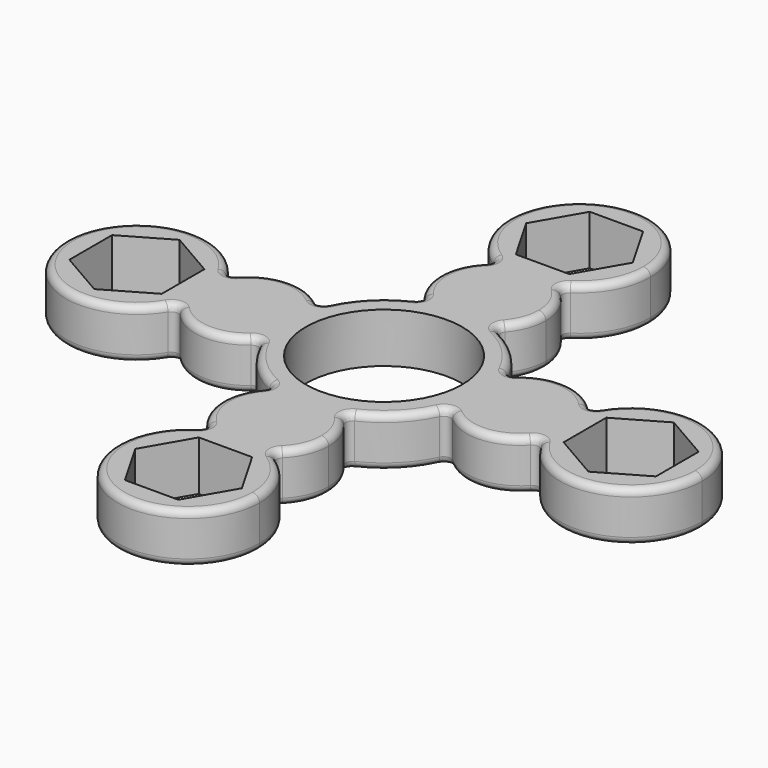
from build123d import *

# Parameters (mm, degrees)
F0_R     = 11
F1_DEPTH = 7
F2_F1_R  = 1
F2_F2_R  = 1


with BuildPart() as f1:
    # F0 (on Top) → F1 (new body)
    with BuildSketch(Plane.XY):
        with BuildLine():
            ThreePointArc((13.2109175103, -4.6337521011), (13.8013195953, -2.3502292287), (14, 0))
            ThreePointArc((14, 0), (13.8013195953, 2.3502292287), (13.2109175103, 4.6337521011))
            ThreePointArc((13.2109175103, 4.6337521011), (11.6082339734, 0), (13.2109175103, -4.6337521011))
        make_face()
        with BuildLine():
            ThreePointArc((13.2109175103, 4.6337521011), (13.8013195953, 2.3502292287), (14, 0))
            ThreePointArc((14, 0), (13.8013195953, -2.3502292287), (13.2109175103, -4.6337521011))
            ThreePointArc((13.2109175103, -4.6337521011), (19.5943342941, -7.4842305201), (25.5553991453, -3.8319787638))
            ThreePointArc((25.5553991453, -3.8319787638), (24.7920618951, 0), (25.5553991453, 3.8319787638))
            ThreePointArc((25.5553991453, 3.8319787638), (19.5943342941, 7.4842305201), (13.2109175103, 4.6337521011))
        make_face()
        with BuildLine():
            ThreePointArc((13.2109175103, -4.6337521011), (11.6082339734, 0), (13.2109175103, 4.6337521011))
            ThreePointArc((13.2109175103, 4.6337521011), (9.8975116316, 9.9014778444), (4.6284588018, 13.2127729535))
            ThreePointArc((4.6284588018, 13.2127729535), (0, 11.6142447293), (-4.6284588018, 13.2127729535))
            ThreePointArc((-4.6284588018, 13.2127729535), (-9.8975116316, 9.9014778444), (-13.2109175103, 4.6337521011))
            ThreePointArc((-13.2109175103, 4.6337521011), (-12.0202203774, 2.4515430373), (-11.6082339734, 0))
            ThreePointArc((-11.6082339734, 0), (-12.0202203774, -2.4515430373), (-13.2109175103, -4.6337521011))
            ThreePointArc((-13.2109175103, -4.6337521011), (-9.8975116316, -9.9014778444), (-4.6284588018, -13.2127729535))
            ThreePointArc((-4.6284588018, -13.2127729535), (0, -11.6142447293), (4.6284588018, -13.2127729535))
            ThreePointArc((4.6284588018, -13.2127729535), (9.8975116316, -9.9014778444), (13.2109175103, -4.6337521011))
        make_face()
        Circle(F0_R, mode=Mode.SUBTRACT)
        with BuildLine():
            ThreePointArc((-4.6284588018, 13.2127729535), (0, 11.6142447293), (4.6284588018, 13.2127729535))
            ThreePointArc((4.6284588018, 13.2127729535), (0, 14), (-4.6284588018, 13.2127729535))
        make_face()
        with BuildLine():
            ThreePointArc((-4.6284588018, 13.2127729535), (0, 14), (4.6284588018, 13.2127729535))
            ThreePointArc((4.6284588018, 13.2127729535), (6.7440136793, 15.8327390545), (7.5, 19.1142447293))
            ThreePointArc((7.5, 19.1142447293), (6.6241857963, 22.6313689147), (4.2012899905, 25.3270671487))
            ThreePointArc((4.2012899905, 25.3270671487), (0, 24.4017110765), (-4.2012899905, 25.3270671487))
            ThreePointArc((-4.2012899905, 25.3270671487), (-7.4953416797, 19.3785421075), (-4.6284588018, 13.2127729535))
        make_face()
        with BuildLine():
            ThreePointArc((44.7920618951, 0), (36.745696009, 9.8073092002), (25.5553991453, 3.8319787638))
            ThreePointArc((25.5553991453, 3.8319787638), (26.3402371118, 1.9869903385), (26.6082339734, 0))
            ThreePointArc((26.6082339734, 0), (26.3402371118, -1.9869903385), (25.5553991453, -3.8319787638))
            ThreePointArc((25.5553991453, -3.8319787638), (36.745696009, -9.8073092002), (44.7920618951, 0))
        make_face()
        Polygon((34.7920618951, 7.5055534995), (41.2920618951, 3.7527767497), (41.2920618951, -3.7527767497), (34.7920618951, -7.5055534995), (28.2920618951, -3.7527767497), (28.2920618951, 3.7527767497), align=None, mode=Mode.SUBTRACT)
        with BuildLine():
            ThreePointArc((26.6082339734, 0), (26.3402371118, 1.9869903385), (25.5553991453, 3.8319787638))
            ThreePointArc((25.5553991453, 3.8319787638), (24.7920618951, 0), (25.5553991453, -3.8319787638))
            ThreePointArc((25.5553991453, -3.8319787638), (26.3402371118, -1.9869903385), (26.6082339734, 0))
        make_face()
        with BuildLine():
            ThreePointArc((7.5, -19.1142447293), (6.7440136793, -15.8327390545), (4.6284588018, -13.2127729535))
            ThreePointArc((4.6284588018, -13.2127729535), (0, -14), (-4.6284588018, -13.2127729535))
            ThreePointArc((-4.6284588018, -13.2127729535), (-7.4953416797, -19.3785421075), (-4.2012899905, -25.3270671487))
            ThreePointArc((-4.2012899905, -25.3270671487), (0, -24.4017110765), (4.2012899905, -25.3270671487))
            ThreePointArc((4.2012899905, -25.3270671487), (6.6241857963, -22.6313689147), (7.5, -19.1142447293))
        make_face()
        with BuildLine():
            ThreePointArc((-4.6284588018, -13.2127729535), (0, -14), (4.6284588018, -13.2127729535))
            ThreePointArc((4.6284588018, -13.2127729535), (0, -11.6142447293), (-4.6284588018, -13.2127729535))
        make_face()
        with BuildLine():
            ThreePointArc((-11.6082339734, 0), (-12.0202203774, 2.4515430373), (-13.2109175103, 4.6337521011))
            ThreePointArc((-13.2109175103, 4.6337521011), (-14, 0), (-13.2109175103, -4.6337521011))
            ThreePointArc((-13.2109175103, -4.6337521011), (-12.0202203774, -2.4515430373), (-11.6082339734, 0))
        make_face()
        with BuildLine():
            ThreePointArc((-13.2109175103, -4.6337521011), (-14, 0), (-13.2109175103, 4.6337521011))
            ThreePointArc((-13.2109175103, 4.6337521011), (-19.5943342941, 7.4842305201), (-25.5553991453, 3.8319787638))
            ThreePointArc((-25.5553991453, 3.8319787638), (-24.9847526949, 1.9536341139), (-24.7920618951, 0))
            ThreePointArc((-24.7920618951, 0), (-24.9847526949, -1.9536341139), (-25.5553991453, -3.8319787638))
            ThreePointArc((-25.5553991453, -3.8319787638), (-19.5943342941, -7.4842305201), (-13.2109175103, -4.6337521011))
        make_face()
        with BuildLine():
            ThreePointArc((10, 34.4017110765), (-5.3845659108, 42.8282435753), (-4.2012899905, 25.3270671487))
            ThreePointArc((-4.2012899905, 25.3270671487), (0, 26.6142447293), (4.2012899905, 25.3270671487))
            ThreePointArc((4.2012899905, 25.3270671487), (8.4265324988, 29.0171451657), (10, 34.4017110765))
        make_face()
        Polygon((-7.5055534995, 34.4017110765), (-3.7527767497, 40.9017110765), (3.7527767497, 40.9017110765), (7.5055534995, 34.4017110765), (3.7527767497, 27.9017110765), (-3.7527767497, 27.9017110765), align=None, mode=Mode.SUBTRACT)
        with BuildLine():
            ThreePointArc((4.2012899905, 25.3270671487), (0, 26.6142447293), (-4.2012899905, 25.3270671487))
            ThreePointArc((-4.2012899905, 25.3270671487), (0, 24.4017110765), (4.2012899905, 25.3270671487))
        make_face()
        with BuildLine():
            ThreePointArc((4.2012899905, -25.3270671487), (0, -24.4017110765), (-4.2012899905, -25.3270671487))
            ThreePointArc((-4.2012899905, -25.3270671487), (0, -26.6142447293), (4.2012899905, -25.3270671487))
        make_face()
        with BuildLine():
            ThreePointArc((4.2012899905, -25.3270671487), (0, -26.6142447293), (-4.2012899905, -25.3270671487))
            ThreePointArc((-4.2012899905, -25.3270671487), (-5.3845659108, -42.8282435753), (10, -34.4017110765))
            ThreePointArc((10, -34.4017110765), (8.4265324988, -29.0171451657), (4.2012899905, -25.3270671487))
        make_face()
        Polygon((-3.7527767497, -27.9017110765), (3.7527767497, -27.9017110765), (7.5055534995, -34.4017110765), (3.7527767497, -40.9017110765), (-3.7527767497, -40.9017110765), (-7.5055534995, -34.4017110765), align=None, mode=Mode.SUBTRACT)
        with BuildLine():
            ThreePointArc((-24.7920618951, 0), (-24.9847526949, 1.9536341139), (-25.5553991453, 3.8319787638))
            ThreePointArc((-25.5553991453, 3.8319787638), (-26.6082339734, 0), (-25.5553991453, -3.8319787638))
            ThreePointArc((-25.5553991453, -3.8319787638), (-24.9847526949, -1.9536341139), (-24.7920618951, 0))
        make_face()
        with BuildLine():
            ThreePointArc((-25.5553991453, -3.8319787638), (-26.6082339734, 0), (-25.5553991453, 3.8319787638))
            ThreePointArc((-25.5553991453, 3.8319787638), (-44.7920618951, 0), (-25.5553991453, -3.8319787638))
        make_face()
        Polygon((-28.2920618951, 3.7527767497), (-28.2920618951, -3.7527767497), (-34.7920618951, -7.5055534995), (-41.2920618951, -3.7527767497), (-41.2920618951, 3.7527767497), (-34.7920618951, 7.5055534995), align=None, mode=Mode.SUBTRACT)
    extrude(amount=F1_DEPTH)

    # F2: fillet of radius 1 on 32 edges, made by hand

    # F2_f1
    f2_f1_edges = [f1.edges().sort_by_distance(p)[0] for p in [
        (-25.5553991453, -3.8319787638, 3.5),
        (-13.2109175103, -4.6337521011, 3.5),
        (4.2012899905, -25.3270671487, 3.5),
        (4.6284588018, -13.2127729535, 3.5),
        (-13.2109175103, 4.6337521011, 3.5),
        (-25.5553991453, 3.8319787638, 3.5),
        (-4.2012899905, 25.3270671487, 3.5),
        (-4.6284588018, 13.2127729535, 3.5),
        (4.6284588018, 13.2127729535, 3.5),
        (4.2012899905, 25.3270671487, 3.5),
        (25.5553991453, 3.8319787638, 3.5),
        (13.2109175103, 4.6337521011, 3.5),
        (13.2109175103, -4.6337521011, 3.5),
        (25.5553991453, -3.8319787638, 3.5),
        (-4.6284588018, -13.2127729535, 3.5),
        (-4.2012899905, -25.3270671487, 3.5),
    ]]
    fillet(f2_f1_edges, radius=F2_F1_R)

    # F2_f2
    f2_f2_edges = [f1.edges().sort_by_distance(p)[0] for p in [
        (-19.5583661198, -7.4864798838, 0),
        (-19.5583661198, -7.4864798838, 7),
        (7.494201041, -19.4091188657, 0),
        (7.494201041, -19.4091188657, 7),
        (-19.5583661198, 7.4864798838, 0),
        (-19.5583661198, 7.4864798838, 7),
        (-7.494201041, 19.4091188657, 0),
        (-7.494201041, 19.4091188657, 7),
        (7.494201041, 19.4091188657, 0),
        (7.494201041, 19.4091188657, 7),
        (19.5583661198, 7.4864798838, 0),
        (19.5583661198, 7.4864798838, 7),
        (19.5583661198, -7.4864798838, 0),
        (19.5583661198, -7.4864798838, 7),
        (-7.494201041, -19.4091188657, 0),
        (-7.494201041, -19.4091188657, 7),
        (-5.449536708, -13.3469740621, 7),
        (-4.9765254333, -25.2658995614, 7),
        (-5.449536708, -13.3469740621, 0),
        (-4.9765254333, -25.2658995614, 0),
        (13.345034304, -5.4532620952, 7),
        (25.4915068246, -4.7241872995, 7),
        (13.345034304, -5.4532620952, 0),
        (25.4915068246, -4.7241872995, 0),
        (25.4915068246, 4.7241872995, 7),
        (13.345034304, 5.4532620952, 7),
        (25.4915068246, 4.7241872995, 0),
        (13.345034304, 5.4532620952, 0),
        (5.449536708, 13.3469740621, 7),
        (4.9765254333, 25.2658995614, 7),
        (5.449536708, 13.3469740621, 0),
        (4.9765254333, 25.2658995614, 0),
        (-4.9765254333, 25.2658995614, 7),
        (-5.449536708, 13.3469740621, 7),
        (-4.9765254333, 25.2658995614, 0),
        (-5.449536708, 13.3469740621, 0),
        (-13.345034304, 5.4532620952, 7),
        (-25.4915068246, 4.7241872995, 7),
        (-13.345034304, 5.4532620952, 0),
        (-25.4915068246, 4.7241872995, 0),
        (4.9765254333, -25.2658995614, 7),
        (5.449536708, -13.3469740621, 7),
        (4.9765254333, -25.2658995614, 0),
        (5.449536708, -13.3469740621, 0),
        (-25.4915068246, -4.7241872995, 7),
        (-13.345034304, -5.4532620952, 7),
        (-25.4915068246, -4.7241872995, 0),
        (-13.345034304, -5.4532620952, 0),
    ]]
    fillet(f2_f2_edges, radius=F2_F2_R)


solid = f1.part
